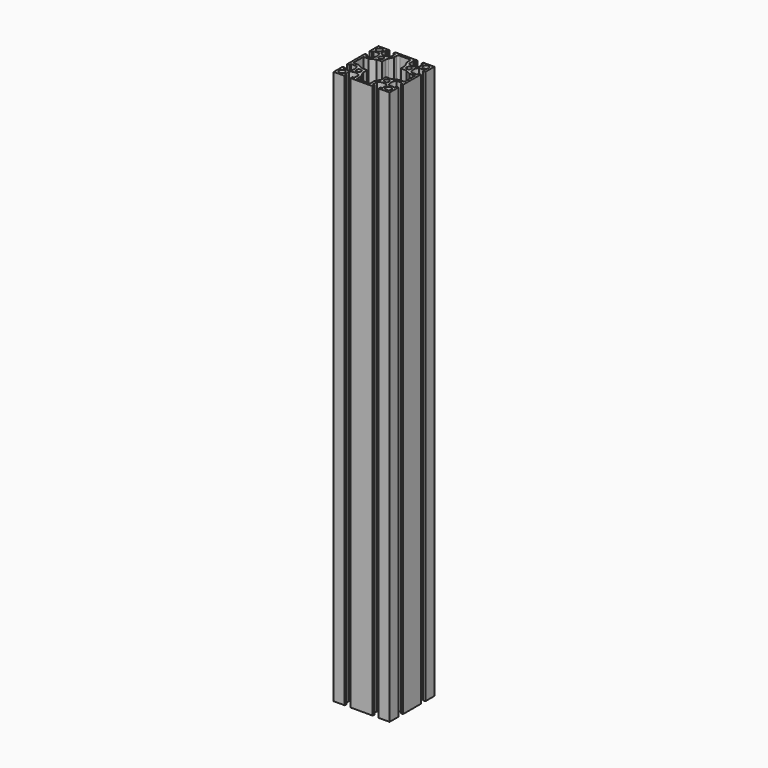
from build123d import *

# Parameters (mm, degrees)
F0_R     = 3
F0_R_2   = 2.5
F1_DEPTH = 595
F2_R     = 2
F3_R     = 7


# Not quite as in the source:
# - a feature names something its author has since deleted; it is built from what else it names


with BuildPart() as f1:
    # F0 (on Top) → F1 (new body)
    with BuildSketch(Plane.XY):
        with BuildLine():
            Line((18.15, -30), (30, -30))
            Line((30, -30), (30, -18.15))
            Line((30, -18.15), (27.5, -18.15))
            Line((27.5, -18.15), (27.5, -20.15))
            Line((27.5, -20.15), (21.5477069044, -20.15))
            ThreePointArc((21.5477069044, -20.15), (19.5, -15), (21.5477069044, -9.85))
            Line((21.5477069044, -9.85), (27.5, -9.85))
            Line((27.5, -9.85), (27.5, -11.85))
            Line((27.5, -11.85), (30, -11.85))
            Line((30, -11.85), (30, 11.85))
            Line((30, 11.85), (27.5, 11.85))
            Line((27.5, 11.85), (27.5, 9.85))
            Line((27.5, 9.85), (21.5477069044, 9.85))
            ThreePointArc((21.5477069044, 9.85), (19.5, 15), (21.5477069044, 20.15))
            Line((21.5477069044, 20.15), (27.5, 20.15))
            Line((27.5, 20.15), (27.5, 18.15))
            Line((27.5, 18.15), (30, 18.15))
            Line((30, 18.15), (30, 30))
            Line((30, 30), (18.15, 30))
            Line((18.15, 30), (18.15, 27.5))
            Line((18.15, 27.5), (20.15, 27.5))
            Line((20.15, 27.5), (20.15, 21.5477069044))
            ThreePointArc((20.15, 21.5477069044), (15, 19.5), (9.85, 21.5477069044))
            Line((9.85, 21.5477069044), (9.85, 27.5))
            Line((9.85, 27.5), (11.85, 27.5))
            Line((11.85, 27.5), (11.85, 30))
            Line((11.85, 30), (-11.85, 30))
            Line((-11.85, 30), (-11.85, 27.5))
            Line((-11.85, 27.5), (-9.85, 27.5))
            Line((-9.85, 27.5), (-9.85, 21.5477069044))
            ThreePointArc((-9.85, 21.5477069044), (-15, 19.5), (-20.15, 21.5477069044))
            Line((-20.15, 21.5477069044), (-20.15, 27.5))
            Line((-20.15, 27.5), (-18.15, 27.5))
            Line((-18.15, 27.5), (-18.15, 30))
            Line((-18.15, 30), (-30, 30))
            Line((-30, 30), (-30, 18.15))
            Line((-30, 18.15), (-27.5, 18.15))
            Line((-27.5, 18.15), (-27.5, 20.15))
            Line((-27.5, 20.15), (-21.5477069044, 20.15))
            ThreePointArc((-21.5477069044, 20.15), (-19.5, 15), (-21.5477069044, 9.85))
            Line((-21.5477069044, 9.85), (-27.5, 9.85))
            Line((-27.5, 9.85), (-27.5, 11.85))
            Line((-27.5, 11.85), (-30, 11.85))
            Line((-30, 11.85), (-30, -11.85))
            Line((-30, -11.85), (-27.5, -11.85))
            Line((-27.5, -11.85), (-27.5, -9.85))
            Line((-27.5, -9.85), (-21.5477069044, -9.85))
            ThreePointArc((-21.5477069044, -9.85), (-19.5, -15), (-21.5477069044, -20.15))
            Line((-21.5477069044, -20.15), (-27.5, -20.15))
            Line((-27.5, -20.15), (-27.5, -18.15))
            Line((-27.5, -18.15), (-30, -18.15))
            Line((-30, -18.15), (-30, -30))
            Line((-30, -30), (-18.15, -30))
            Line((-18.15, -30), (-18.15, -27.5))
            Line((-18.15, -27.5), (-20.15, -27.5))
            Line((-20.15, -27.5), (-20.15, -21.5477069044))
            ThreePointArc((-20.15, -21.5477069044), (-15, -19.5), (-9.85, -21.5477069044))
            Line((-9.85, -21.5477069044), (-9.85, -27.5))
            Line((-9.85, -27.5), (-11.85, -27.5))
            Line((-11.85, -27.5), (-11.85, -30))
            Line((-11.85, -30), (11.85, -30))
            Line((11.85, -30), (11.85, -27.5))
            Line((11.85, -27.5), (9.85, -27.5))
            Line((9.85, -27.5), (9.85, -21.5477069044))
            ThreePointArc((9.85, -21.5477069044), (15, -19.5), (20.15, -21.5477069044))
            Line((20.15, -21.5477069044), (20.15, -27.5))
            Line((20.15, -27.5), (18.15, -27.5))
            Line((18.15, -27.5), (18.15, -30))
        make_face()
        with Locations((-25, -25)):
            Circle(F0_R, mode=Mode.SUBTRACT)
        with Locations((-15, -15)):
            Circle(F0_R_2, mode=Mode.SUBTRACT)
        with Locations((25, -25)):
            Circle(F0_R, mode=Mode.SUBTRACT)
        with Locations((15, -15)):
            Circle(F0_R_2, mode=Mode.SUBTRACT)
        with Locations((-25, 25)):
            Circle(F0_R, mode=Mode.SUBTRACT)
        with Locations((-15, 15)):
            Circle(F0_R_2, mode=Mode.SUBTRACT)
        Polygon((-7, 22), (-7, 27.5), (0, 27.5), (7, 27.5), (7, 22), (10, 16), (10, 10), (16, 10), (22, 7), (27.5, 7), (27.5, 0), (27.5, -7), (22, -7), (16, -10), (10, -10), (10, -16), (7, -22), (7, -27.5), (0, -27.5), (-7, -27.5), (-7, -22), (-10, -16), (-10, -10), (-16, -10), (-22, -7), (-27.5, -7), (-27.5, 0), (-27.5, 7), (-22, 7), (-16, 10), (-10, 10), (-10, 16), align=None, mode=Mode.SUBTRACT)
        with Locations((15, 15)):
            Circle(F0_R_2, mode=Mode.SUBTRACT)
        with Locations((25, 25)):
            Circle(F0_R, mode=Mode.SUBTRACT)
    extrude(amount=F1_DEPTH)

    # F2
    f2_edges = [f1.edges().sort_by_distance(p)[0] for p in [
        (-7, 27.5, 297.5),
        (7, 27.5, 297.5),
    ]]
    fillet(f2_edges, radius=F2_R)

    # F3
    f3_edges = [f1.edges().sort_by_distance(p)[0] for p in [
        (-10, 16, 297.5),
        (10, 16, 297.5),
    ]]
    fillet(f3_edges, radius=F3_R)


solid = f1.part
